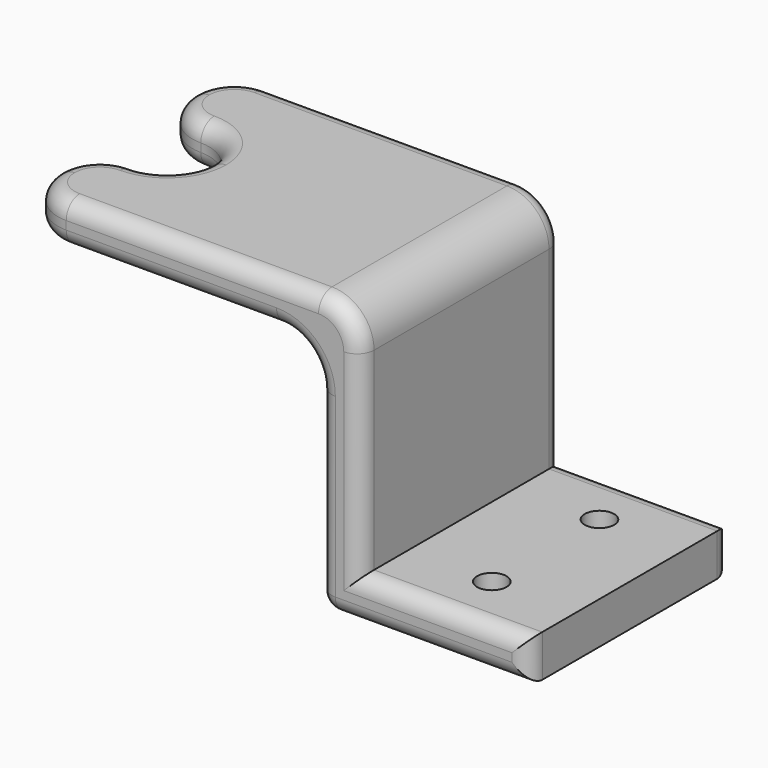
from build123d import *

# Parameters (mm, degrees)
F0_W      = 40
F0_H      = 30
F1_DEPTH  = 5
F2_W      = 10
F2_H      = 10
F3_DEPTH  = 25
F4_W      = 5
F4_H      = 30
F5_DEPTH  = 28
F6_W      = 30
F6_H      = 5
F7_DEPTH  = 20
F8_R      = 4.99999
F9_R      = 2
F10_R     = 1.75
F11_DEPTH = 25


# Not quite as in the source:
# - a fillet or chamfer is up to 0.001 mm smaller than in the source, because OpenCascade refuses the exact size


with BuildPart() as f1:
    # F0 (on Top) → F1 (new body)
    with BuildSketch(Plane.XY):
        Rectangle(F0_W, F0_H)
    extrude(amount=F1_DEPTH)

    # F2 (on face) → F3 (cut)
    with BuildSketch(Plane.XY.offset(5)):
        with Locations((-15, 0)):
            Rectangle(F2_W, F2_H)
    extrude(amount=-F3_DEPTH, mode=Mode.SUBTRACT)

    # F4 (on face) → F5 (join)
    with BuildSketch(Plane(origin=(0, 0, 0), x_dir=(1, 0, 0), z_dir=(0, 0, -1))):
        with Locations((17.5, 0)):
            Rectangle(F4_W, F4_H)
    extrude(amount=F5_DEPTH)

    # F6 (on face) → F7 (join)
    with BuildSketch(Plane.YZ.offset(20)):
        with Locations((0, -25.5)):
            Rectangle(F6_W, F6_H)
    extrude(amount=F7_DEPTH)

    # F8 (radius 5 in the source; OpenCascade refuses exactly that, so slightly less here)
    f8_edges = [f1.edges().sort_by_distance(p)[0] for p in [
        (-20, 5, 2.5),
        (-20, -5, 2.5),
        (-20, -15, 2.5),
        (-20, 15, 2.5),
        (20, 0, 5),
        (-10, -5, 2.5),
        (-10, 5, 2.5),
        (15, 0, 0),
    ]]
    fillet(f8_edges, radius=F8_R)

    # F9
    f9_edges = [f1.edges().sort_by_distance(p)[0] for p in [
        (0, -15, 5),
        (-18.535537, -13.535537, 5),
        (15.00001, 0, 5),
        (-20, -10, 5),
        (0, 15, 5),
        (-18.535537, -6.464463, 5),
        (-18.535537, 13.535537, 5),
        (-15, -5, 5),
        (-20, 10, 5),
        (-11.464463, -3.535537, 5),
        (-18.535537, 6.464463, 5),
        (-10, 0, 5),
        (-15, 5, 5),
        (-11.464463, 3.535537, 5),
        (15, -15, -16.499995),
        (15, 0, -28),
        (-15.00001, -15, 2.5),
        (18.535537, -15, 3.535537),
        (-2.5, -15, 0),
        (20, -15, -11.499995),
        (13.535537, -15, -1.464463),
        (30, -15, -23),
        (40, -15, -25.5),
        (27.5, -15, -28),
        (20, 15, -11.499995),
        (18.535537, 15, 3.535537),
        (30, 15, -23),
        (40, 15, -25.5),
        (-15.00001, 15, 2.5),
        (27.5, 15, -28),
        (-2.5, 15, 0),
        (15, 15, -16.499995),
        (13.535537, 15, -1.464463),
    ]]
    fillet(f9_edges, radius=F9_R)

    # F10 (on face) → F11 (cut)
    with BuildSketch(Plane.XY.offset(-23)):
        with Locations((30, -8)):
            Circle(F10_R)
        with Locations((30, 8)):
            Circle(F10_R)
    extrude(amount=-F11_DEPTH, mode=Mode.SUBTRACT)


solid = f1.part
